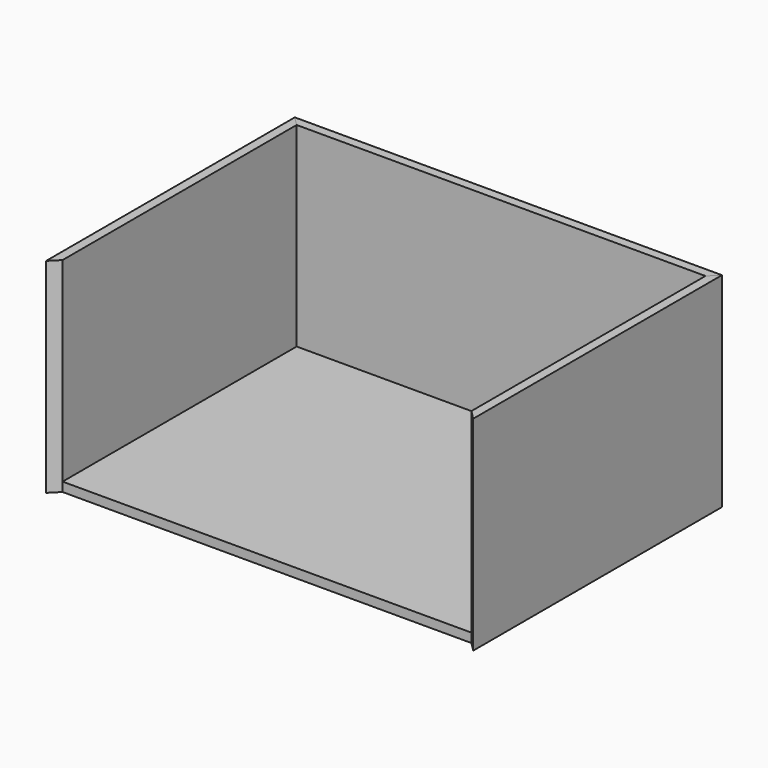
from build123d import *

# Parameters (mm, degrees)
F1_W      = 556.26
F1_H      = 265.938
F2_DEPTH  = 11.938
F3_W      = 532.384
F3_H      = 381
F4_DEPTH  = 11.938
F5_W      = 404.876
F5_H      = 265.938
F6_DEPTH  = 11.938
F8_SIZE   = 11.93799
F8_2_SIZE = 11.93799
F8_3_SIZE = 11.93799


# Not quite as in the source:
# - a variable given as a bare number and used for a length is read in inches; the dataset says mm whatever the document's units were
# - a fillet or chamfer is up to 0.001 mm smaller than in the source, because OpenCascade refuses the exact size


with BuildPart() as f2:
    # F1 (on Front) → F2 (new body)
    with BuildSketch(Plane.XZ):
        with Locations((0, 132.969)):
            Rectangle(F1_W, F1_H)
    extrude(amount=F2_DEPTH)

    # F8 (size 11.938 in the source; OpenCascade refuses exactly that, so slightly less here)
    f8_edges = [f2.edges().sort_by_distance(p)[0] for p in [
        (278.13, -11.938, 132.969),
        (-278.13, -11.938, 132.969),
    ]]
    chamfer(f8_edges, length=F8_SIZE)


with BuildPart() as f4:
    # F3 (on face) → F4 (new body)
    with BuildSketch(Plane(origin=(0, 0, 0), x_dir=(1, 0, 0), z_dir=(0, 0, -1))):
        with Locations((0, 202.438)):
            Rectangle(F3_W, F3_H)
    extrude(amount=-F4_DEPTH)


with BuildPart() as f6:
    # F5 (on face) → F6 (new body)
    with BuildSketch(Plane(origin=(-266.192, 0, 0), x_dir=(0, -1, 0), z_dir=(-1, 0, 0))):
        with Locations((202.438, 132.969)):
            Rectangle(F5_W, F5_H)
    extrude(amount=F6_DEPTH)


with BuildPart() as f7_1:
    # F7: instance of F6
    add(f6.part.mirror(Plane.YZ))

    # F8#2 (size 11.938 in the source; OpenCascade refuses exactly that, so slightly less here)
    f8_2_edges = [f7_1.edges().sort_by_distance(p)[0] for p in [
        (266.192, 0, 132.969),
        (266.192, -404.876, 132.969),
    ]]
    chamfer(f8_2_edges, length=F8_2_SIZE)


with BuildPart() as f6_1:
    add(f6.part)

    # F8#3 (size 11.938 in the source; OpenCascade refuses exactly that, so slightly less here)
    f8_3_edges = [f6_1.edges().sort_by_distance(p)[0] for p in [
        (-266.192, 0, 132.969),
        (-266.192, -404.876, 132.969),
    ]]
    chamfer(f8_3_edges, length=F8_3_SIZE)


solid = Compound([f2.part, f4.part, f7_1.part, f6_1.part])
